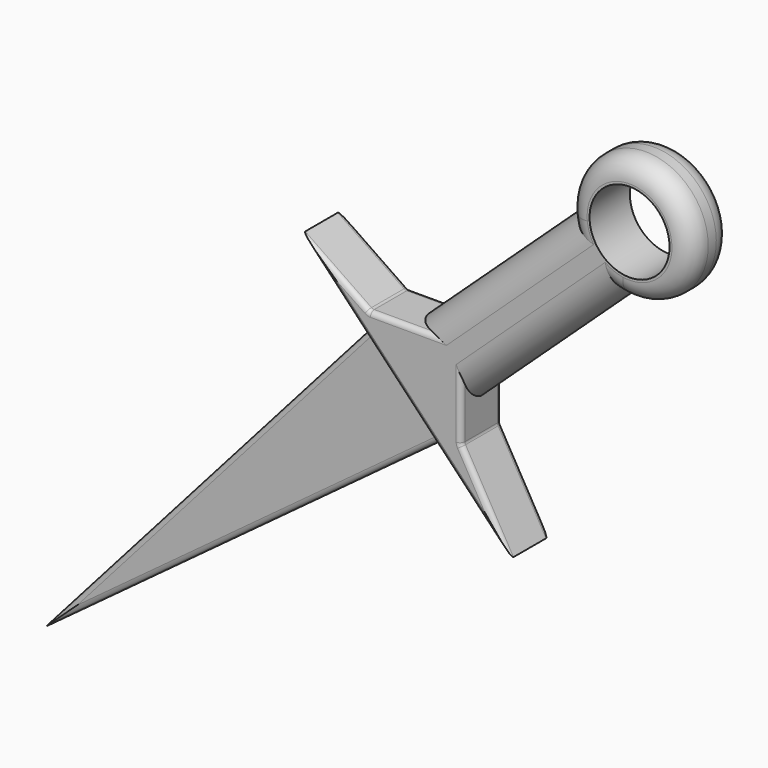
from build123d import *

# Parameters (mm, degrees)
F1_DEPTH     = 12.7
F3_START     = 4.064
F3_DEPTH     = 3.81
F4_T4_DEPTH  = 93.1383939159
F4_S5_R      = 15.7806026061
F4_T6_DEPTH  = 52
F4_T11_DEPTH = 93.1383939159
F4_S12_R     = 15.7806026061
F4_T13_DEPTH = 52
F4_T18_DEPTH = 92.8850738108
F4_S20_R     = 15.7806026061
F4_T21_DEPTH = 52
F4_T25_DEPTH = 92.8850738108
F4_S27_R     = 15.7806026061
F4_T28_DEPTH = 52
F5_R         = 5.07999
F6_R         = 1.2264204897
F7_R         = 1.27
F8_R         = 1.27
F9_R         = 10.0844220232
F10_DEPTH    = 12.7


# Not quite as in the source:
# - a fillet or chamfer that OpenCascade refuses, or shapes differently, is made with other operations: its cross-section is extruded or revolved along the edge and cut away or added
# - a fillet or chamfer is up to 0.001 mm smaller than in the source, because OpenCascade refuses the exact size


with BuildPart() as f1:
    # F0 (on Front) → F1 (new body)
    with BuildSketch(Plane.XZ):
        with BuildLine():
            Line((13.2145041692, 58.2067854702), (-3.8163531803, 69.8823442173))
            Line((-3.8163531803, 69.8823442173), (48.701737076, 14.6710211411))
            Line((48.701737076, 14.6710211411), (36.4542003432, 35.9734042756))
            Line((36.4542003432, 35.9734042756), (36.4542003432, 44.2807382619))
            Line((36.4542003432, 44.2807382619), (76.6045332289, 81.554791994))
            ThreePointArc((76.6045332289, 81.554791994), (67.4885852958, 86.3005665919), (63.228149501, 95.6531902927))
            Line((63.228149501, 95.6531902927), (22.8921659291, 58.2067854702))
            Line((22.8921659291, 58.2067854702), (13.2145041692, 58.2067854702))
        make_face()
        with BuildLine():
            ThreePointArc((94.7170448112, 97.1621498466), (78.1810966455, 112.9246646109), (63.228149501, 95.6531902927))
            ThreePointArc((63.228149501, 95.6531902927), (67.4885852958, 86.3005665919), (76.6045332289, 81.554791994))
            ThreePointArc((76.6045332289, 81.554791994), (89.2376190734, 85.207520043), (94.7170448112, 97.1621498466))
        make_face()
    extrude(amount=F1_DEPTH)

    # F4: fillet of radius 7.62 on 4 edges, made by hand


with BuildPart() as f3:
    # F2 (on Front) → F3 (new body)
    with BuildSketch(Plane.XZ.offset(F3_START)):
        Polygon((11.5275448188, 53.340408951), (-72.9976892471, -42.2478355467), (30.2482489496, 34.0428091586), align=None)
    extrude(amount=F3_DEPTH)

    # F7
    f7_edges = [f3.edges().sort_by_distance(p)[0] for p in [
        (-21.37472, -7.874, -4.102513),
        (-30.735072, -7.874, 5.546287),
    ]]
    fillet(f7_edges, radius=F7_R)

    # F8
    f8_edges = [f3.edges().sort_by_distance(p)[0] for p in [
        (-30.735072, -4.064, 5.546287),
        (-21.37472, -4.064, -4.102513),
    ]]
    fillet(f8_edges, radius=F8_R)


with BuildPart() as f4_tool2:
    # F4_s3 → F4_t4 (new body)
    with BuildSketch(Plane(origin=(95.6156726243, 0, 88.7659818207), x_dir=(0, 1, 0), z_dir=(-0.7328699241, 0, -0.6803687782))):
        with BuildLine():
            ThreePointArc((-5.08, -27.0828874864), (-10.4681536726, -24.8510411591), (-12.7, -19.4628874864))
            Line((-12.7, -19.4628874864), (-12.7, -27.0828874864))
            Line((-12.7, -27.0828874864), (-5.08, -27.0828874864))
        make_face()
    extrude(amount=F4_T4_DEPTH)

    # F4_s5 → F4_t6 (cut, symmetric)
    with BuildSketch(Plane.XZ.offset(8.9)):
        with Locations((78.936442205, 97.1621498466)):
            Circle(F4_S5_R)
    extrude(amount=F4_T6_DEPTH, both=True, mode=Mode.SUBTRACT)

    split(bisect_by=Plane.XY.offset(58.2067854702), keep=Keep.TOP)


with BuildPart() as f1_1:
    add(f1.part)

    # F4_t1: cut F4_tool2
    add(f4_tool2.part, mode=Mode.SUBTRACT)


with BuildPart() as f4_tool9:
    # F4_s10 → F4_t11 (new body)
    with BuildSketch(Plane(origin=(95.6156726243, 0, 88.7659818207), x_dir=(0, 1, 0), z_dir=(-0.7328699241, 0, -0.6803687782))):
        with BuildLine():
            ThreePointArc((-7.62, -27.0828874864), (-2.2318463274, -24.8510411591), (0, -19.4628874864))
            Line((0, -19.4628874864), (0, -27.0828874864))
            Line((0, -27.0828874864), (-7.62, -27.0828874864))
        make_face()
    extrude(amount=F4_T11_DEPTH)

    # F4_s12 → F4_t13 (cut, symmetric)
    with BuildSketch(Plane.XZ.offset(3.8)):
        with Locations((78.936442205, 97.1621498466)):
            Circle(F4_S12_R)
    extrude(amount=F4_T13_DEPTH, both=True, mode=Mode.SUBTRACT)

    split(bisect_by=Plane.XY.offset(58.2067854702), keep=Keep.TOP)


with BuildPart() as f1_2:
    add(f1_1.part)

    # F4_t8: cut F4_tool9
    add(f4_tool9.part, mode=Mode.SUBTRACT)


with BuildPart() as f4_tool16:
    # F4_s17 → F4_t18 (new body)
    with BuildSketch(Plane(origin=(27.6976599878, 0, 25.7134621917), x_dir=(0, 1, 0), z_dir=(0.7328699241, 0, 0.6803687782))):
        with BuildLine():
            ThreePointArc((-5.08, 7.6497215416), (-10.4681536726, 9.8815678689), (-12.7, 15.2697215416))
            Line((-12.7, 15.2697215416), (-12.7, 7.6497215416))
            Line((-12.7, 7.6497215416), (-5.08, 7.6497215416))
        make_face()
    extrude(amount=F4_T18_DEPTH)

    split(bisect_by=Plane.YZ.offset(36.4542003432), keep=Keep.TOP)

    # F4_s20 → F4_t21 (cut, symmetric)
    with BuildSketch(Plane.XZ.offset(8.9)):
        with Locations((78.936442205, 97.1621498466)):
            Circle(F4_S20_R)
    extrude(amount=F4_T21_DEPTH, both=True, mode=Mode.SUBTRACT)


with BuildPart() as f1_3:
    add(f1_2.part)

    # F4_t15: cut F4_tool16
    add(f4_tool16.part, mode=Mode.SUBTRACT)


with BuildPart() as f4_tool23:
    # F4_s24 → F4_t25 (new body)
    with BuildSketch(Plane(origin=(27.6976599878, 0, 25.7134621917), x_dir=(0, 1, 0), z_dir=(0.7328699241, 0, 0.6803687782))):
        with BuildLine():
            ThreePointArc((-7.62, 7.6497215416), (-2.2318463274, 9.8815678689), (0, 15.2697215416))
            Line((0, 15.2697215416), (0, 7.6497215416))
            Line((0, 7.6497215416), (-7.62, 7.6497215416))
        make_face()
    extrude(amount=F4_T25_DEPTH)

    split(bisect_by=Plane.YZ.offset(36.4542003432), keep=Keep.TOP)

    # F4_s27 → F4_t28 (cut, symmetric)
    with BuildSketch(Plane.XZ.offset(3.8)):
        with Locations((78.936442205, 97.1621498466)):
            Circle(F4_S27_R)
    extrude(amount=F4_T28_DEPTH, both=True, mode=Mode.SUBTRACT)


with BuildPart() as f1_4:
    add(f1_3.part)

    # F4_t22: cut F4_tool23
    add(f4_tool23.part, mode=Mode.SUBTRACT)

    # F5 (radius 5.08 in the source; OpenCascade refuses exactly that, so slightly less here)
    f5_edges = [f1_4.edges().sort_by_distance(p)[0] for p in [
        (87.15426, 0, 110.634154),
        (87.15426, -12.7, 110.634154),
    ]]
    fillet(f5_edges, radius=F5_R)

    # F6
    f6_edges = [f1_4.edges().sort_by_distance(p)[0] for p in [
        (4.699075, 0, 64.044565),
        (23.653239, 0, 58.206785),
        (4.699075, -12.7, 64.044565),
        (23.653239, -12.7, 58.206785),
        (36.4542, 0, 45.325811),
        (42.577969, 0, 25.322213),
        (36.4542, -12.7, 45.325811),
        (42.577969, -12.7, 25.322213),
        (36.4542, -6.35, 35.973404),
        (13.214504, -6.35, 58.206785),
        (22.442692, 0, 42.276683),
        (22.442692, -12.7, 42.276683),
    ]]
    fillet(f6_edges, radius=F6_R)

    # F9 (on face) → F10 (cut)
    with BuildSketch(Plane.XZ.offset(12.7)):
        with Locations((78.936442205, 97.1621498466)):
            Circle(F9_R)
    extrude(amount=-F10_DEPTH, mode=Mode.SUBTRACT)


solid = Compound([f3.part, f1_4.part])
